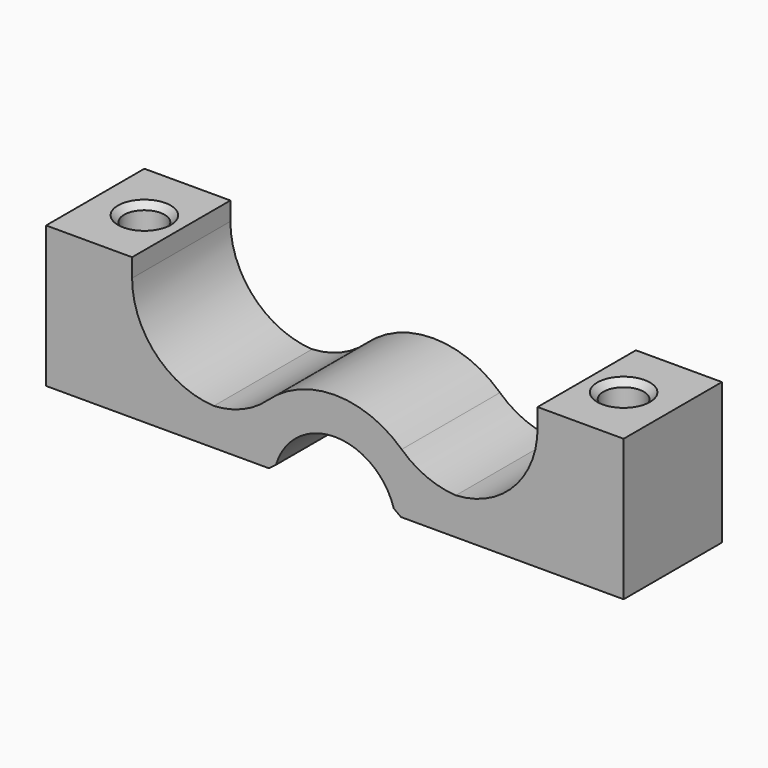
from build123d import *

# Parameters (mm, degrees)
F1_DEPTH    = 5
F2_T1_DEPTH = 5
F2_T3_DEPTH = 5
F3_T1_DEPTH = 6.2324692544
F3_T3_DEPTH = 6.2324692544
F4_R        = 1.65
F5_DEPTH    = 11.501
F6_SIZE     = 0.5


# Not quite as in the source:
# - a fillet or chamfer that OpenCascade refuses, or shapes differently, is made with other operations: its cross-section is extruded or revolved along the edge and cut away or added
# - a pattern or mirror of a feature is missing from the dataset's text; its kind, count and spacing are read off the source's solid


with BuildPart() as f1:
    # F0 (on Front) → F1 (new body, symmetric)
    with BuildSketch(Plane.XZ):
        with BuildLine():
            Line((4.8989794856, 1), (23.5, 1))
            Line((23.5, 1), (23.5, 12.5))
            Line((23.5, 12.5), (16.5, 12.5))
            Line((16.5, 12.5), (16.5, 4))
            Line((16.5, 4), (6.9282032303, 4))
            ThreePointArc((6.9282032303, 4), (4, 6.9282032303), (0, 8))
            ThreePointArc((0, 8), (-4, 6.9282032303), (-6.9282032303, 4))
            Line((-6.9282032303, 4), (-16.5, 4))
            Line((-16.5, 4), (-16.5, 12.5))
            Line((-16.5, 12.5), (-23.5, 12.5))
            Line((-23.5, 12.5), (-23.5, 1))
            Line((-23.5, 1), (-4.8989794856, 1))
            ThreePointArc((-4.8989794856, 1), (-3.1622776602, 3.8729833462), (0, 5))
            ThreePointArc((0, 5), (3.1622776602, 3.8729833462), (4.8989794856, 1))
        make_face()
    extrude(amount=F1_DEPTH, both=True)

    # F2: fillet of radius 7 on 8 edges, made by hand

    # F2_s2 → F2_t1 (join)
    with BuildSketch(Plane.XZ.offset(-5)):
        with BuildLine():
            ThreePointArc((16.5, 11), (14.4497474683, 6.0502525317), (9.5, 4))
            Line((9.5, 4), (16.5, 4))
            Line((16.5, 4), (16.5, 11))
        make_face()
        with BuildLine():
            ThreePointArc((10.1980390272, 4), (7.6420004255, 4.4833546462), (5.4389541478, 5.8666666667))
            ThreePointArc((5.4389541478, 5.8666666667), (6.2536194731, 4.989212712), (6.9282032303, 4))
            Line((6.9282032303, 4), (10.1980390272, 4))
        make_face()
        with BuildLine():
            ThreePointArc((-5.4389541478, 5.8666666667), (-7.6420004255, 4.4833546462), (-10.1980390272, 4))
            Line((-10.1980390272, 4), (-6.9282032303, 4))
            ThreePointArc((-6.9282032303, 4), (-6.2536194731, 4.989212712), (-5.4389541478, 5.8666666667))
        make_face()
        with BuildLine():
            ThreePointArc((-9.5, 4), (-14.4497474683, 6.0502525317), (-16.5, 11))
            Line((-16.5, 11), (-16.5, 4))
            Line((-16.5, 4), (-9.5, 4))
        make_face()
    extrude(amount=F2_T1_DEPTH)

    # F2_s4 → F2_t3 (join)
    with BuildSketch(Plane.XZ):
        with BuildLine():
            ThreePointArc((16.5, 11), (14.4497474683, 6.0502525317), (9.5, 4))
            Line((9.5, 4), (16.5, 4))
            Line((16.5, 4), (16.5, 11))
        make_face()
        with BuildLine():
            ThreePointArc((10.1980390272, 4), (7.6420004255, 4.4833546462), (5.4389541478, 5.8666666667))
            ThreePointArc((5.4389541478, 5.8666666667), (6.2536194731, 4.989212712), (6.9282032303, 4))
            Line((6.9282032303, 4), (10.1980390272, 4))
        make_face()
        with BuildLine():
            ThreePointArc((-5.4389541478, 5.8666666667), (-7.6420004255, 4.4833546462), (-10.1980390272, 4))
            Line((-10.1980390272, 4), (-6.9282032303, 4))
            ThreePointArc((-6.9282032303, 4), (-6.2536194731, 4.989212712), (-5.4389541478, 5.8666666667))
        make_face()
        with BuildLine():
            ThreePointArc((-9.5, 4), (-14.4497474683, 6.0502525317), (-16.5, 11))
            Line((-16.5, 11), (-16.5, 4))
            Line((-16.5, 4), (-9.5, 4))
        make_face()
    extrude(amount=F2_T3_DEPTH)

    # F3: chamfer of 0.5 on 4 edges, made by hand

    # F3_s2 → F3_t1 (cut)
    with BuildSketch(Plane.XZ.offset(-6.2324692544)):
        with BuildLine():
            Line((-4.7731743681, 1.4483837223), (-5.3918225964, 0.9880608955))
            Line((-5.3918225964, 0.9880608955), (-5.3918225964, 0.9780608955))
            ThreePointArc((-5.3918225964, 0.9780608955), (-5.145401041, 0.99), (-4.8989794856, 0.99))
            Line((-4.8989794856, 0.99), (-4.8891815266, 0.998))
            ThreePointArc((-4.8891815266, 0.998), (-4.8374189809, 1.2245315852), (-4.7635959284, 1.445510833))
            Line((-4.7635959284, 1.445510833), (-4.7731743681, 1.4483837223))
        make_face()
        with BuildLine():
            Line((4.7731743681, 1.4483837223), (5.3918225964, 0.9880608955))
            Line((5.3918225964, 0.9880608955), (5.3918225964, 0.9780608955))
            ThreePointArc((5.3918225964, 0.9780608955), (5.145401041, 0.99), (4.8989794856, 0.99))
            Line((4.8989794856, 0.99), (4.8891815266, 0.998))
            ThreePointArc((4.8891815266, 0.998), (4.8374189809, 1.2245315852), (4.7635959284, 1.445510833))
            Line((4.7635959284, 1.445510833), (4.7731743681, 1.4483837223))
        make_face()
    extrude(amount=F3_T1_DEPTH, mode=Mode.SUBTRACT)

    # F3_s4 → F3_t3 (cut)
    with BuildSketch(Plane.XZ):
        with BuildLine():
            Line((-4.7731743681, 1.4483837223), (-5.3918225964, 0.9880608955))
            Line((-5.3918225964, 0.9880608955), (-5.3918225964, 0.9780608955))
            ThreePointArc((-5.3918225964, 0.9780608955), (-5.145401041, 0.99), (-4.8989794856, 0.99))
            Line((-4.8989794856, 0.99), (-4.8891815266, 0.998))
            ThreePointArc((-4.8891815266, 0.998), (-4.8374189809, 1.2245315852), (-4.7635959284, 1.445510833))
            Line((-4.7635959284, 1.445510833), (-4.7731743681, 1.4483837223))
        make_face()
        with BuildLine():
            Line((4.7731743681, 1.4483837223), (5.3918225964, 0.9880608955))
            Line((5.3918225964, 0.9880608955), (5.3918225964, 0.9780608955))
            ThreePointArc((5.3918225964, 0.9780608955), (5.145401041, 0.99), (4.8989794856, 0.99))
            Line((4.8989794856, 0.99), (4.8891815266, 0.998))
            ThreePointArc((4.8891815266, 0.998), (4.8374189809, 1.2245315852), (4.7635959284, 1.445510833))
            Line((4.7635959284, 1.445510833), (4.7731743681, 1.4483837223))
        make_face()
    extrude(amount=F3_T3_DEPTH, mode=Mode.SUBTRACT)

    # F4 (on face) → F5 (cut, through all)
    with BuildSketch(Plane.XY.offset(12.5)):
        with Locations((19.5, 0)):
            Circle(F4_R)
    f5 = extrude(amount=-F5_DEPTH, mode=Mode.SUBTRACT)

    # F5_copies: F5 across plane
    add(f5.mirror(Plane(origin=(0, 0, 0), x_dir=(0, 0, -1), z_dir=(-1, 0, 0))), mode=Mode.SUBTRACT)

    # F6
    f6_edges = [f1.edges().sort_by_distance(p)[0] for p in [
        (19.5, 1.65, 12.5),
        (19.5, -1.65, 12.5),
        (19.5, 1.65, 1),
        (-19.5, 1.65, 1),
        (-19.5, 1.65, 12.5),
        (19.5, -1.65, 1),
        (-19.5, -1.65, 1),
        (-19.5, -1.65, 12.5),
    ]]
    chamfer(f6_edges, length=F6_SIZE)


solid = f1.part
